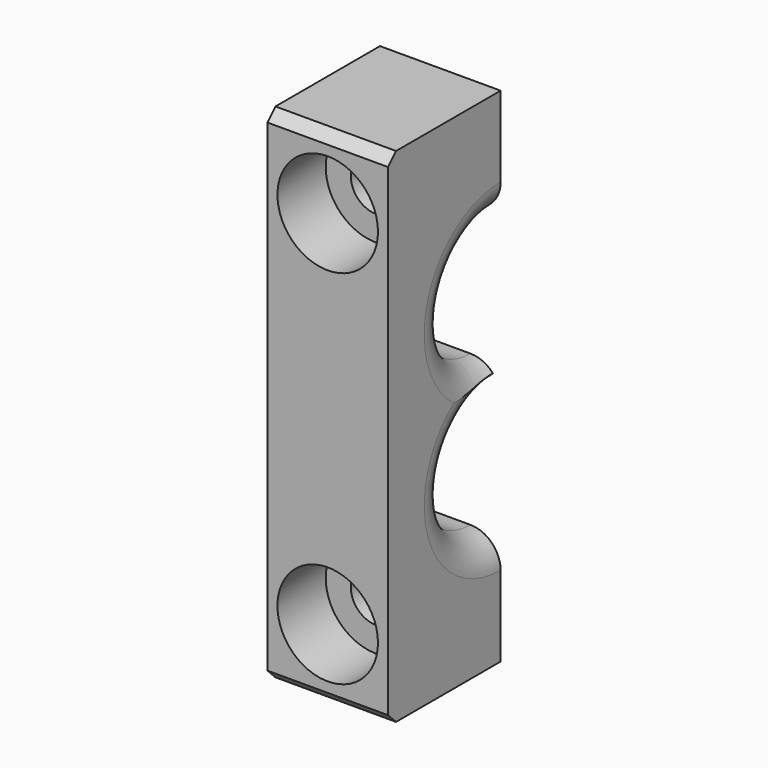
from build123d import *

# Parameters (mm, degrees)
F0_W      = 12
F0_H      = 50
F1_DEPTH  = 30
F2_R      = 6.5
F3_DEPTH  = 12.001
F4_W      = 20
F4_H      = 50
F5_DEPTH  = 2
F8_D      = 5
F9_W      = 10
F9_H      = 20
F10_DEPTH = 8
F11_R     = 5
F12_DEPTH = 6
F13_SIZE  = 1
F15_W     = 41.8421067297
F15_H     = 67.5000026822
F16_DEPTH = 25


# Not quite as in the source:
# - a fillet or chamfer that OpenCascade refuses, or shapes differently, is made with other operations: its cross-section is extruded or revolved along the edge and cut away or added


with BuildPart() as f1:
    # F0 (on Front) → F1 (new body)
    with BuildSketch(Plane.XZ):
        Rectangle(F0_W, F0_H)
    extrude(amount=F1_DEPTH)

    # F2 (on face) → F3 (cut, through all)
    with BuildSketch(Plane.YZ.offset(6)):
        with Locations((-16, 7.5)):
            Circle(F2_R)
        with Locations((-16, -7.5)):
            Circle(F2_R)
    extrude(amount=-F3_DEPTH, mode=Mode.SUBTRACT)

    # F4 (on Front) → F5 (join)
    with BuildSketch(Plane.XZ):
        Rectangle(F4_W, F4_H)
    extrude(amount=F5_DEPTH)

    # F6: fillet of radius 3 on 4 edges, made by hand

    # F6_s1 → F6_t2 (revolve, cut)
    with BuildSketch(Plane.XY.offset(7.5)):
        with BuildLine():
            ThreePointArc((-6, -6.5), (-5.1213203436, -8.6213203436), (-3, -9.5))
            Line((-3, -9.5), (-6, -9.5))
            Line((-6, -9.5), (-6, -6.5))
        make_face()
    revolve(axis=Axis((-6, -16, 7.5), (1, 0, 0)), mode=Mode.SUBTRACT)

    # F6_s3 → F6_t4 (revolve, cut)
    with BuildSketch(Plane.XY.offset(-7.5)):
        with BuildLine():
            ThreePointArc((-6, -6.5), (-5.1213203436, -8.6213203436), (-3, -9.5))
            Line((-3, -9.5), (-6, -9.5))
            Line((-6, -9.5), (-6, -6.5))
        make_face()
    revolve(axis=Axis((-6, -16, -7.5), (1, 0, 0)), mode=Mode.SUBTRACT)

    # F6_s5 → F6_t6 (revolve, cut)
    with BuildSketch(Plane.XY.offset(7.5)):
        with BuildLine():
            ThreePointArc((3, -9.5), (5.1213203436, -8.6213203436), (6, -6.5))
            Line((6, -6.5), (6, -9.5))
            Line((6, -9.5), (3, -9.5))
        make_face()
    revolve(axis=Axis((6, -16, 7.5), (1, 0, 0)), mode=Mode.SUBTRACT)

    # F6_s7 → F6_t8 (revolve, cut)
    with BuildSketch(Plane.XY.offset(-7.5)):
        with BuildLine():
            ThreePointArc((3, -9.5), (5.1213203436, -8.6213203436), (6, -6.5))
            Line((6, -6.5), (6, -9.5))
            Line((6, -9.5), (3, -9.5))
        make_face()
    revolve(axis=Axis((6, -16, -7.5), (1, 0, 0)), mode=Mode.SUBTRACT)

    # F8 (through all)
    with Locations(Plane(origin=(0, 0, 0), x_dir=(-1, 0, 0), z_dir=(0, 1, 0))):
        with Locations((0, 18), (0, -18)):
            Hole(F8_D / 2)

    # F9 (on face) → F10 (cut)
    with BuildSketch(Plane(origin=(0, 0, 0), x_dir=(-1, 0, 0), z_dir=(0, 1, 0))):
        Polygon((0, 12.1110272543), (5.1, 15.0555136271), (5.1, 20.9444863729), (0, 23.8889727457), (-5.1, 20.9444863729), (-5.1, 15.0555136271), align=None)
        Rectangle(F9_W, F9_H)
        Polygon((5.1, -20.9444863729), (5.1, -15.0555136271), (0, -12.1110272543), (-5.1, -15.0555136271), (-5.1, -20.9444863729), (0, -23.8889727457), align=None)
    extrude(amount=-F10_DEPTH, mode=Mode.SUBTRACT)

    # F11 (on face) → F12 (cut)
    with BuildSketch(Plane.XZ.offset(30)):
        with Locations((0, 18)):
            Circle(F11_R)
        with Locations((0, -18)):
            Circle(F11_R)
    extrude(amount=-F12_DEPTH, mode=Mode.SUBTRACT)

    # F13
    f13_edges = [f1.edges().sort_by_distance(p)[0] for p in [
        (0, -30, -25),
        (0, -30, 25),
    ]]
    chamfer(f13_edges, length=F13_SIZE)

    # F15 (on offset) → F16 (cut)
    with BuildSketch(Plane.XZ.offset(16)):
        with Locations((-0.493420288, -0.09868294)):
            Rectangle(F15_W, F15_H)
    extrude(amount=-F16_DEPTH, mode=Mode.SUBTRACT)


solid = f1.part
